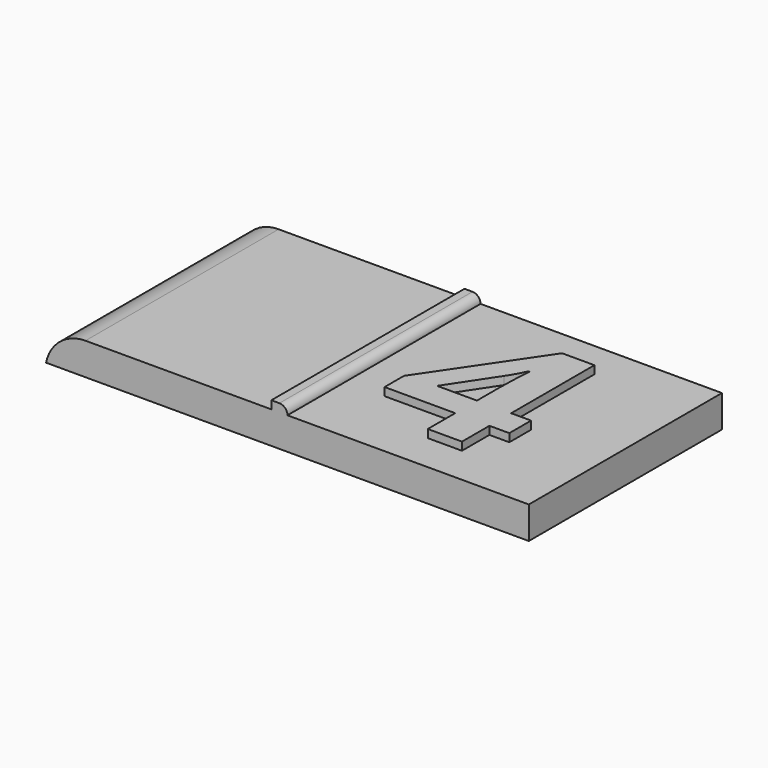
from build123d import *

# Parameters (mm, degrees)
F0_W         = 60
F0_H         = 30
F1_DEPTH     = 4
F2_W         = 2
F2_H         = 30
F3_DEPTH     = 1
F4_R         = 0.99999
F5_TEXT_SIZE = 28.8201948731
F6_DEPTH     = 1
F7_T1_DEPTH  = 54.4948974279


# Not quite as in the source:
# - a fillet or chamfer that OpenCascade refuses, or shapes differently, is made with other operations: its cross-section is extruded or revolved along the edge and cut away or added
# - a fillet or chamfer is up to 0.001 mm smaller than in the source, because OpenCascade refuses the exact size
# - Text() gives the source's letters only with a copy of the font that has no kerning and outlines rounded to 1/6400 em; it was checked with that copy


with BuildPart() as f1:
    # F0 (on Top) → F1 (new body)
    with BuildSketch(Plane.XY):
        with Locations((30, 15)):
            Rectangle(F0_W, F0_H)
    extrude(amount=F1_DEPTH)

    # F2 (on face) → F3 (join)
    with BuildSketch(Plane.XY.offset(4)):
        with Locations((29, 15)):
            Rectangle(F2_W, F2_H)
    extrude(amount=F3_DEPTH)

    # F4 (radius 1 in the source; OpenCascade refuses exactly that, so slightly less here)
    f4_edges = [f1.edges().sort_by_distance(p)[0] for p in [
        (30, 15, 5),
    ]]
    fillet(f4_edges, radius=F4_R)

    # F5 (on face) → F6 (join)
    with BuildSketch(Plane.XY.offset(4)):
        with Locations((34.3574509025, 4.7624194995)):
            Text('4', F5_TEXT_SIZE, font='Open Sans', font_style=FontStyle.BOLD, text_align=(TextAlign.LEFT, TextAlign.BOTTOM))
    extrude(amount=F6_DEPTH)

    # F7: fillet of radius 5 on 1 edges, made by hand

    # F7_s2 → F7_t1 (cut)
    with BuildSketch(Plane.XZ.offset(-42.2474487139)):
        with BuildLine():
            ThreePointArc((4.8989794856, 4), (1.7367018254, 2.8729833462), (0, 0))
            Line((0, 0), (0, 4))
            Line((0, 4), (4.8989794856, 4))
        make_face()
    extrude(amount=F7_T1_DEPTH, mode=Mode.SUBTRACT)


solid = f1.part
